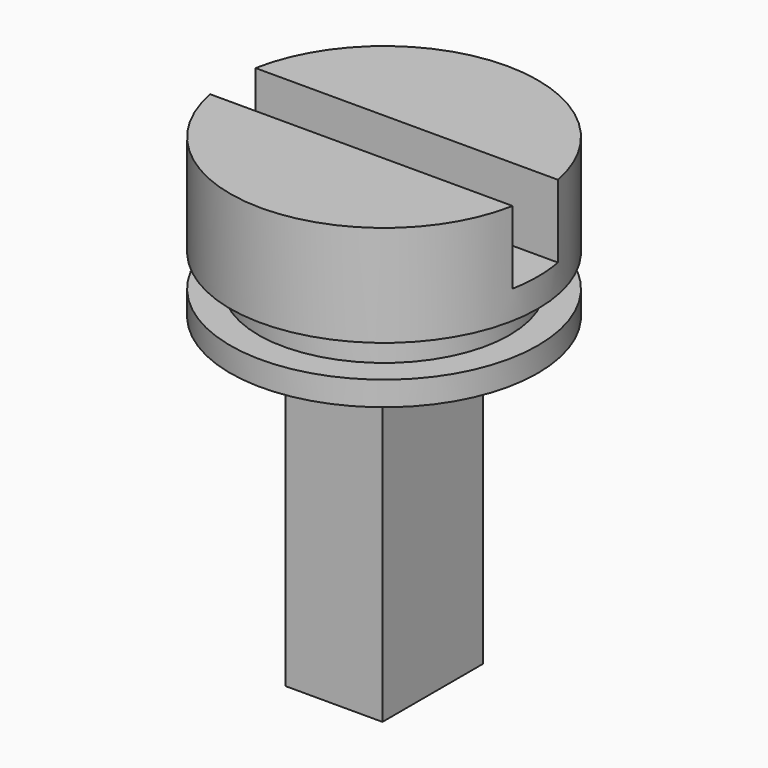
from build123d import *

# Parameters (mm, degrees)
F0_R     = 4.826
F1_DEPTH = 3.175
F2_W     = 11.9897948747
F2_H     = 1.778
F3_DEPTH = 2.286
F4_R     = 3.937
F5_DEPTH = 1.016
F6_R     = 4.826
F7_DEPTH = 0.762
F8_W     = 3.048
F8_H     = 3.937
F9_DEPTH = 9.906


# Not quite as in the source:
# - the program builds the solid bodies; features that only make, move or delete a surface that nothing else refers to are left out


with BuildPart() as f1:
    # F0 (on Top) → F1 (new body)
    with BuildSketch(Plane.XY):
        Circle(F0_R)
    extrude(amount=-F1_DEPTH)

    # F2 (on face) → F3 (cut)
    with BuildSketch(Plane.XY):
        Rectangle(F2_W, F2_H)
    extrude(amount=-F3_DEPTH, mode=Mode.SUBTRACT)

    # F4 (on face) → F5 (join)
    with BuildSketch(Plane(origin=(0, 0, -3.175), x_dir=(1, 0, 0), z_dir=(0, 0, -1))):
        Circle(F4_R)
    extrude(amount=F5_DEPTH)

    # F6 (on face) → F7 (join)
    with BuildSketch(Plane(origin=(0, 0, -4.191), x_dir=(1, 0, 0), z_dir=(0, 0, -1))):
        Circle(F6_R)
    extrude(amount=F7_DEPTH)

    # F8 (on face) → F9 (join)
    with BuildSketch(Plane(origin=(0, 0, -4.953), x_dir=(1, 0, 0), z_dir=(0, 0, -1))):
        Rectangle(F8_W, F8_H)
    extrude(amount=F9_DEPTH)


solid = f1.part
